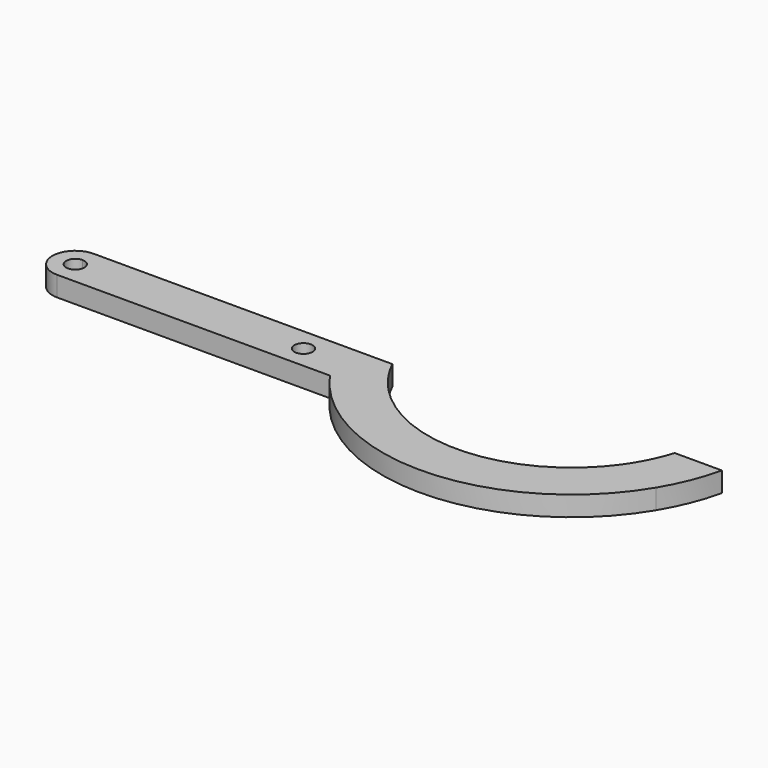
from build123d import *

# Parameters (mm, degrees)
F1_DEPTH = 3.5
F3_DEPTH = 3.501


# Not quite as in the source:
# - a feature names something its author has since deleted; it is built from what else it names


with BuildPart() as f1:
    # F0 (on Top) → F1 (new body)
    with BuildSketch(Plane.XY):
        with BuildLine():
            ThreePointArc((-50, 4), (-54, 0), (-50, -4))
            Line((-50, -4), (-50, 4))
        make_face()
        with BuildLine():
            Line((-50, 4), (-50, -4))
            ThreePointArc((-50, -4), (-47.1715728753, -2.8284271247), (-46, 0))
            ThreePointArc((-46, 0), (-47.1715728753, 2.8284271247), (-50, 4))
        make_face()
        with BuildLine():
            Line((-50, -4), (-2.1705369066, -4))
            ThreePointArc((-2.1705369066, -4), (-4.496147737, -0.1398594601), (-6.2767977228, 4))
            Line((-6.2767977228, 4), (-50, 4))
            ThreePointArc((-50, 4), (-47.1715728753, 2.8284271247), (-46, 0))
            ThreePointArc((-46, 0), (-47.1715728753, -2.8284271247), (-50, -4))
        make_face()
        with BuildLine():
            Line((-2.1705369066, -4), (8.5147968103, -4))
            ThreePointArc((8.5147968103, -4), (6.5521066164, -2.1007939556), (4.8068842373, 0))
            ThreePointArc((4.8068842373, 0), (3.4991426783, 1.9433902318), (2.3778443952, 4))
            Line((2.3778443952, 4), (-6.2767977228, 4))
            ThreePointArc((-6.2767977228, 4), (-4.496147737, -0.1398594601), (-2.1705369066, -4))
        make_face()
        with BuildLine():
            ThreePointArc((53.4299716908, -2.0579830418), (51.9707952498, -3.4807996328), (50, -4))
            Line((50, -4), (41.4852031897, -4))
            ThreePointArc((41.4852031897, -4), (25, -10.1547594742), (8.5147968103, -4))
            Line((8.5147968103, -4), (-2.1705369066, -4))
            ThreePointArc((-2.1705369066, -4), (26.1573251317, -18.1345540838), (53.4299716908, -2.0579830418))
        make_face()
        with BuildLine():
            Line((41.4852031897, -4), (50, -4))
            ThreePointArc((50, -4), (47.1715728753, -2.8284271247), (46, 0))
            Line((46, 0), (45.1931157627, 0))
            ThreePointArc((45.1931157627, 0), (43.4478933836, -2.1007939556), (41.4852031897, -4))
        make_face()
        with BuildLine():
            ThreePointArc((46, 0), (47.1715728753, -2.8284271247), (50, -4))
            Line((50, -4), (50, 0))
            Line((50, 0), (46, 0))
        make_face()
        with BuildLine():
            Line((50, 0), (50, -4))
            ThreePointArc((50, -4), (51.9707952498, -3.4807996328), (53.4299716908, -2.0579830418))
            ThreePointArc((53.4299716908, -2.0579830418), (53.8548597097, -1.0677343389), (54, 0))
            ThreePointArc((54, 0), (52.8284271247, 2.8284271247), (50, 4))
            Line((50, 4), (50, 0))
        make_face()
        with BuildLine():
            Line((46, 0), (50, 0))
            Line((50, 0), (50, 4))
            ThreePointArc((50, 4), (48.0292047387, 3.4807996262), (46.5700282955, 2.0579830189))
            ThreePointArc((46.5700282955, 2.0579830189), (46.1451402867, 1.067734326), (46, 0))
        make_face()
        with BuildLine():
            ThreePointArc((46.5700282955, 2.0579830189), (48.0292047387, 3.4807996262), (50, 4))
            Line((50, 4), (47.6221556048, 4))
            ThreePointArc((47.6221556048, 4), (47.1174170499, 3.0174382017), (46.5700282955, 2.0579830189))
        make_face()
        with BuildLine():
            Line((45.1931157627, 0), (46, 0))
            ThreePointArc((46, 0), (46.1451402867, 1.067734326), (46.5700282955, 2.0579830189))
            ThreePointArc((46.5700282955, 2.0579830189), (45.9069097174, 1.0120390952), (45.1931157627, 0))
        make_face()
        with BuildLine():
            ThreePointArc((54, 0), (53.8548597097, -1.0677343389), (53.4299716908, -2.0579830418))
            ThreePointArc((53.4299716908, -2.0579830418), (55.7469814085, 2.5959196207), (57.3080045365, 7.5548056666))
            Line((57.3080045365, 7.5548056666), (49.0277132816, 7.5548056666))
            ThreePointArc((49.0277132816, 7.5548056666), (48.3925570986, 5.7506650728), (47.6221556048, 4))
            Line((47.6221556048, 4), (50, 4))
            ThreePointArc((50, 4), (52.8284271247, 2.8284271247), (54, 0))
        make_face()
    extrude(amount=F1_DEPTH)

    # F2 (on face) → F3 (cut, through all)
    with BuildSketch(Plane.XY.offset(3.5)):
        with BuildLine():
            ThreePointArc((-48.4, 0), (-48.8686291501, 1.1313708499), (-50, 1.6))
            Line((-50, 1.6), (-50, 0))
            Line((-50, 0), (-48.4, 0))
        make_face()
        with BuildLine():
            Line((-50, 0), (-50, 1.6))
            ThreePointArc((-50, 1.6), (-51.6, 0), (-50, -1.6))
            Line((-50, -1.6), (-50, 0))
        make_face()
        with BuildLine():
            ThreePointArc((-8.4, 0), (-10, 1.6), (-11.6, 0))
            ThreePointArc((-11.6, 0), (-10, -1.6), (-8.4, 0))
        make_face()
        with BuildLine():
            Line((-48.4, 0), (-50, 0))
            Line((-50, 0), (-50, -1.6))
            ThreePointArc((-50, -1.6), (-48.8686291501, -1.1313708499), (-48.4, 0))
        make_face()
    extrude(amount=-F3_DEPTH, mode=Mode.SUBTRACT)


solid = f1.part
